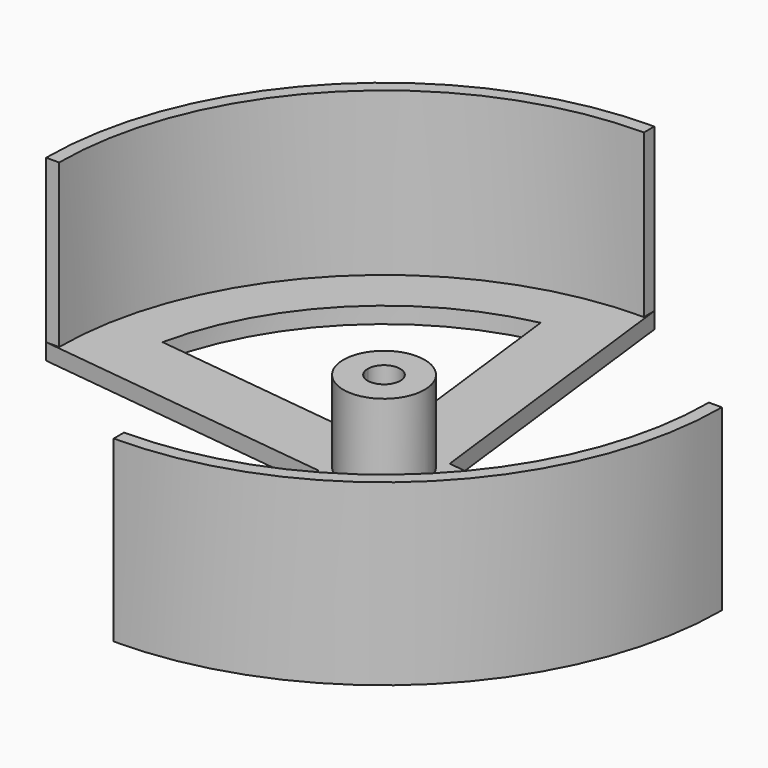
from build123d import *
from build123d import SkipClean  # not in build123d's __all__

# Parameters (mm, degrees)
F1_DEPTH = 10
F2_R     = 1
F3_DEPTH = 1
F4_R     = 2.5
F4_R_2   = 1
F5_DEPTH = 5
F6_COUNT = 2


with BuildPart() as f1:
    # F0 (on Top) → F1 (new body)
    with BuildSketch(Plane.XY):
        with BuildLine():
            ThreePointArc((-20, 0), (-14.1421356237, 14.1421356237), (0, 20))
            Line((0, 20), (0, 20.8))
            ThreePointArc((0, 20.8), (-14.7078210487, 14.7078210487), (-20.8, 0))
            Line((-20.8, 0), (-20, 0))
        make_face()
    extrude(amount=F1_DEPTH)

    # F2 (on Top) → F3 (join)
    with BuildSketch(Plane.XY):
        with BuildLine():
            Line((2.4818765697, 0.3004807692), (0, 20.8))
            ThreePointArc((0, 20.8), (-14.7078210487, 14.7078210487), (-20.8, 0))
            Line((-20.8, 0), (-0.3004807692, -2.4818765697))
            ThreePointArc((-0.3004807692, -2.4818765697), (1.767766953, -1.767766953), (2.4818765697, 0.3004807692))
        make_face()
        Circle(F2_R, mode=Mode.SUBTRACT)
        with BuildLine():
            ThreePointArc((-16.4313102282, 3.5002920141), (-11.8793939239, 11.8793939239), (-3.5002920141, 16.4313102282))
            Line((-3.5002920141, 16.4313102282), (-1.9348109471, 3.5009293908))
            ThreePointArc((-1.9348109471, 3.5009293908), (-2.8284271247, 2.8284271247), (-3.5009293908, 1.9348109471))
            Line((-3.5009293908, 1.9348109471), (-16.4313102282, 3.5002920141))
        make_face(mode=Mode.SUBTRACT)
    extrude(amount=-F3_DEPTH)

    # F4 (on face) → F5 (join)
    with BuildSketch(Plane.XY):
        Circle(F4_R)
        Circle(F4_R_2, mode=Mode.SUBTRACT)
    with SkipClean():  # cleaning this boolean's faces spoils the solid; the shape is the same uncleaned
        extrude(amount=F5_DEPTH)

    # F6: F1 ×2 about axis
    f6_axis = Axis((0, 0, 5), (0, 0, 1))


with BuildPart() as f1_1:
    add(f1.part, clean=False)
    for i in range(1, F6_COUNT):
        add(f1.part.rotate(f6_axis, i * 360 / F6_COUNT), clean=False)


solid = f1_1.part
